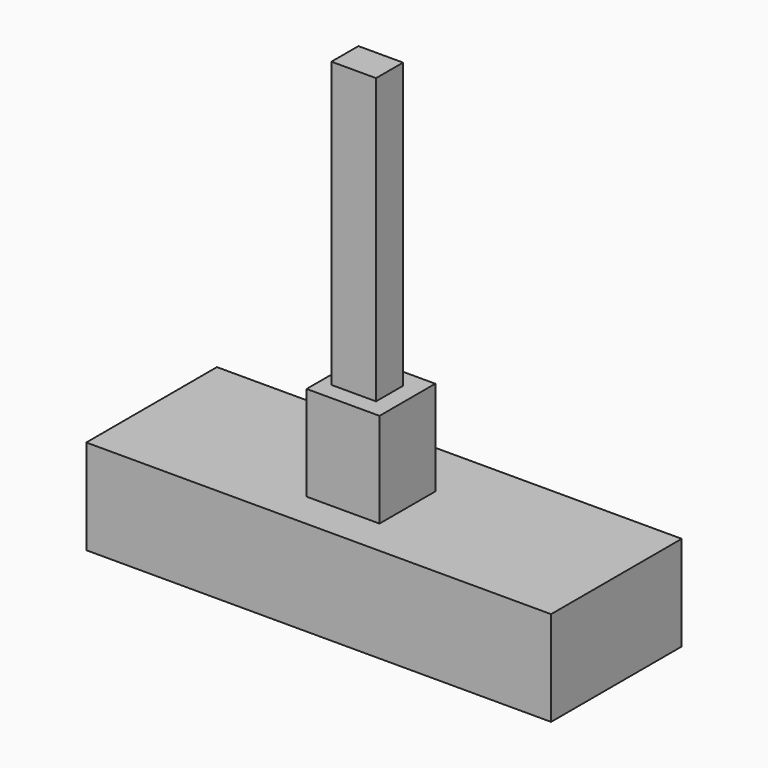
from build123d import *

# Parameters (mm, degrees)
F0_W     = 122.5000061095
F0_H     = 43.0327896029
F1_DEPTH = 25
F2_W     = 19.2213132977
F2_H     = 18.3606566861
F3_DEPTH = 25
F5_W     = 11.7622986436
F5_H     = 8.8934430387
F6_DEPTH = 75


# Not quite as in the source:
# - the program builds the solid bodies; features that only make, move or delete a surface that nothing else refers to are left out


with BuildPart() as f1:
    # F0 (on Top) → F1 (new body)
    with BuildSketch(Plane.XY):
        with Locations((1.8647518009, 3.872952424)):
            Rectangle(F0_W, F0_H)
    extrude(amount=F1_DEPTH)

    # F2 (on face) → F3 (join)
    with BuildSketch(Plane.XY.offset(25)):
        with Locations((0.7172133774, 1.0040984489)):
            Rectangle(F2_W, F2_H)
    extrude(amount=F3_DEPTH)

    # F5 (on face) → F6 (join)
    with BuildSketch(Plane.XY.offset(50)):
        with Locations((-0.1434423029, 0.8606557967)):
            Rectangle(F5_W, F5_H)
    extrude(amount=F6_DEPTH)


solid = f1.part
